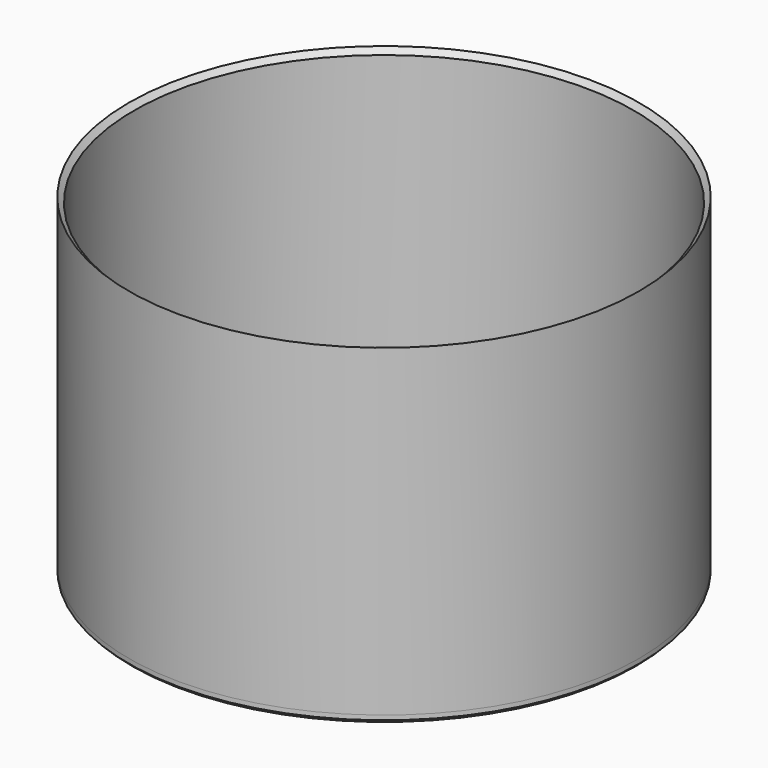
from build123d import *

# Parameters (mm, degrees)
F0_R     = 39.3
F0_R_2   = 38.5
F1_DEPTH = 1.2
F2_DEPTH = 50
F4_SIZE  = 0.5


# Not quite as in the source:
# - a fillet or chamfer that OpenCascade refuses, or shapes differently, is made with other operations: its cross-section is extruded or revolved along the edge and cut away or added


with BuildPart() as f1:
    # F0 (on Top) → F1 (new body)
    with BuildSketch(Plane.XY):
        Circle(F0_R)
        Circle(F0_R_2, mode=Mode.SUBTRACT)
        Circle(F0_R_2)
    extrude(amount=-F1_DEPTH)

    # F0 (on Top) → F2 (join)
    with BuildSketch(Plane.XY):
        Circle(F0_R)
        Circle(F0_R_2, mode=Mode.SUBTRACT)
    extrude(amount=F2_DEPTH)

    # F3: chamfer of 1 on 1 edges, made by hand

    # F3_s1 → F3_t2 (revolve, cut)
    with BuildSketch(Plane.XZ):
        Polygon((39.5, 50), (38.5, 49), (38.5, 50), align=None)
    revolve(axis=Axis((0, 0, 50), (0, 0, 1)), mode=Mode.SUBTRACT)

    # F4
    f4_edges = [f1.edges().sort_by_distance(p)[0] for p in [
        (-39.3, 0, -1.2),
    ]]
    chamfer(f4_edges, length=F4_SIZE)


solid = f1.part
